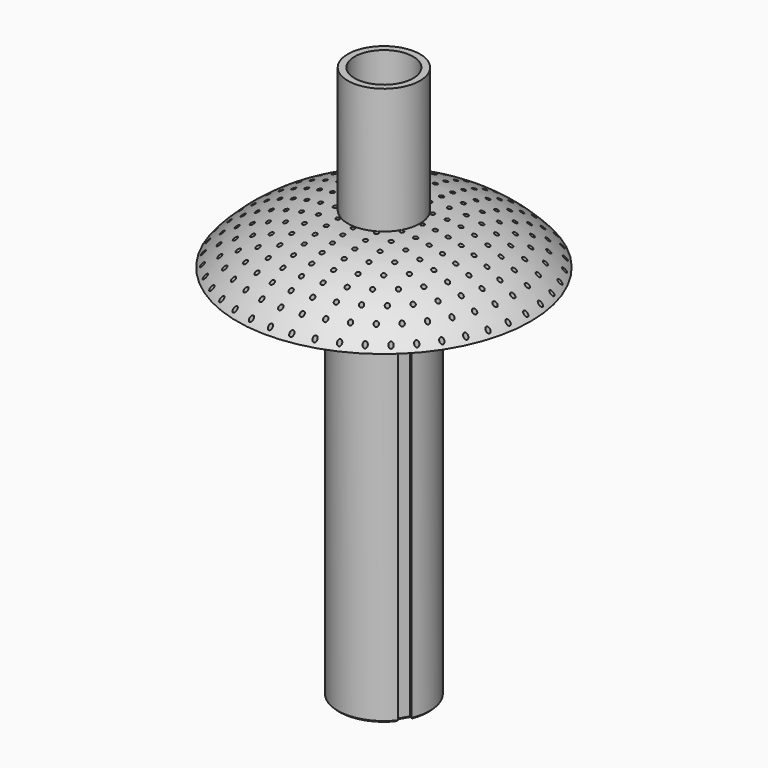
from build123d import *

# Parameters (mm, degrees)
F0_R      = 5.5
F1_DEPTH  = 45
F2_W      = 1.3165529235
F2_H      = 2.0980495028
F3_DEPTH  = 50
F4_R      = 17.5
F5_DEPTH  = 6
F7_R      = 3.5
F8_DEPTH  = 45
F9_SIZE   = 0.2
F11_R     = 0.25
F12_DEPTH = 20.5
F16_DEPTH = 15


# Not quite as in the source:
# - a fillet or chamfer that OpenCascade refuses, or shapes differently, is made with other operations: its cross-section is extruded or revolved along the edge and cut away or added


with BuildPart() as f1:
    # F0 (on Top) → F1 (new body)
    with BuildSketch(Plane.XY):
        Circle(F0_R)
    extrude(amount=F1_DEPTH)

    # F2 (on face) → F3 (cut)
    with BuildSketch(Plane.XY.offset(45)):
        with Locations((0.0565157097, 6.1680867802)):
            Rectangle(F2_W, F2_H)
        Polygon((-4.7906338463, -1.9405028355), (-6.6075980141, -2.9895275869), (-5.9493215523, -4.1296958641), (-4.1323573845, -3.0806711127), align=None)
        Polygon((4.0758416748, -3.1785591934), (5.8928058426, -4.2275839448), (6.5510823044, -3.0874156676), (4.7341181365, -2.0383909162), align=None)
    extrude(amount=-F3_DEPTH, mode=Mode.SUBTRACT)

    # F4 (on face) → F5 (join)
    with BuildSketch(Plane.XY.offset(45)):
        Circle(F4_R)
    extrude(amount=F5_DEPTH)

    # F6: fillet of radius 17.5 on 1 edges, made by hand

    # F6_s1 → F6_t2 (revolve, cut)
    with BuildSketch(Plane.XZ):
        with BuildLine():
            ThreePointArc((17.5, 45), (11.5547824148, 49.4295323221), (4.3090940417, 51))
            Line((4.3090940417, 51), (17.5, 51))
            Line((17.5, 51), (17.5, 45))
        make_face()
    revolve(axis=Axis((0, 0, 51), (0, 0, 1)), mode=Mode.SUBTRACT)

    # F7 (on face) → F8 (cut)
    with BuildSketch(Plane.XY.offset(51)):
        Circle(F7_R)
    extrude(amount=-F8_DEPTH, mode=Mode.SUBTRACT)

    # F9
    f9_edges = [f1.edges().sort_by_distance(p)[0] for p in [
        (4.40498, -2.608475, 0),
        (4.791347, 2.700554, 0),
        (0.714792, 5.286208, 0),
        (0.056516, 5.119062, 0),
        (-0.601761, 5.293022, 0),
        (-4.734422, 2.799151, 0),
        (-4.935387, -2.024076, 0),
        (-4.461496, -2.510587, 0),
        (-4.283011, -3.167651, 0),
        (-0.056925, -5.499705, 0),
        (4.220594, -3.262132, 0),
        (4.884772, -2.125371, 0),
    ]]
    chamfer(f9_edges, length=F9_SIZE)

    # F11 (on offset) → F12 (cut)
    with BuildSketch(Plane.XY.offset(40)):
        with BuildLine():
            ThreePointArc((0, 4.35), (0.1767766953, 4.4232233047), (0.25, 4.6))
            ThreePointArc((0.25, 4.6), (0.1767766953, 4.7767766953), (0, 4.85))
            Line((0, 4.85), (0, 4.35))
        make_face()
        with BuildLine():
            ThreePointArc((0, 6.39), (-0.25, 6.14), (0, 5.89))
            Line((0, 5.89), (0, 6.39))
        make_face()
        with BuildLine():
            Line((0, 6.39), (0, 5.89))
            ThreePointArc((0, 5.89), (0.1767766953, 5.9632233047), (0.25, 6.14))
            ThreePointArc((0.25, 6.14), (0.1767766953, 6.3167766953), (0, 6.39))
        make_face()
        with BuildLine():
            Line((0, 4.35), (0, 4.85))
            ThreePointArc((0, 4.85), (-0.25, 4.6), (0, 4.35))
        make_face()
        with Locations((0, 7.68)):
            Circle(F11_R)
        with Locations((0, 9.22)):
            Circle(F11_R)
        with Locations((0, 10.76)):
            Circle(F11_R)
        with Locations((0, 12.3)):
            Circle(F11_R)
        with Locations((-2.3, 3.9837168574)):
            Circle(F11_R)
        with Locations((-3.9837168574, 2.3)):
            Circle(F11_R)
        with Locations((-4.6, 0)):
            Circle(F11_R)
        with Locations((-3.9837168574, -2.3)):
            Circle(F11_R)
        with Locations((-2.3, -3.9837168574)):
            Circle(F11_R)
        with Locations((0, -4.6)):
            Circle(F11_R)
        with Locations((2.3, -3.9837168574)):
            Circle(F11_R)
        with Locations((3.9837168574, -2.3)):
            Circle(F11_R)
        with Locations((4.6, 0)):
            Circle(F11_R)
        with Locations((3.9837168574, 2.3)):
            Circle(F11_R)
        with Locations((2.3, 3.9837168574)):
            Circle(F11_R)
        with Locations((-2.3496762747, 5.6726203296)):
            Circle(F11_R)
        with Locations((-4.3416356365, 4.3416356365)):
            Circle(F11_R)
        with Locations((-5.6726203296, 2.3496762747)):
            Circle(F11_R)
        with Locations((-6.14, 0)):
            Circle(F11_R)
        with Locations((-5.6726203296, -2.3496762747)):
            Circle(F11_R)
        with Locations((-4.3416356365, -4.3416356365)):
            Circle(F11_R)
        with Locations((-2.3496762747, -5.6726203296)):
            Circle(F11_R)
        with Locations((0, -6.14)):
            Circle(F11_R)
        with Locations((2.3496762747, -5.6726203296)):
            Circle(F11_R)
        with Locations((4.3416356365, -4.3416356365)):
            Circle(F11_R)
        with Locations((5.6726203296, -2.3496762747)):
            Circle(F11_R)
        with Locations((6.14, 0)):
            Circle(F11_R)
        with Locations((5.6726203296, 2.3496762747)):
            Circle(F11_R)
        with Locations((4.3416356365, 4.3416356365)):
            Circle(F11_R)
        with Locations((2.3496762747, 5.6726203296)):
            Circle(F11_R)
        with Locations((-2.3732505168, 7.3041140451)):
            Circle(F11_R)
        with Locations((-4.5141907376, 6.2132505168)):
            Circle(F11_R)
        with Locations((-6.2132505168, 4.5141907376)):
            Circle(F11_R)
        with Locations((-7.3041140451, 2.3732505168)):
            Circle(F11_R)
        with Locations((-7.68, 0)):
            Circle(F11_R)
        with Locations((-7.3041140451, -2.3732505168)):
            Circle(F11_R)
        with Locations((-6.2132505168, -4.5141907376)):
            Circle(F11_R)
        with Locations((-4.5141907376, -6.2132505168)):
            Circle(F11_R)
        with Locations((-2.3732505168, -7.3041140451)):
            Circle(F11_R)
        with Locations((0, -7.68)):
            Circle(F11_R)
        with Locations((2.3732505168, -7.3041140451)):
            Circle(F11_R)
        with Locations((4.5141907376, -6.2132505168)):
            Circle(F11_R)
        with Locations((6.2132505168, -4.5141907376)):
            Circle(F11_R)
        with Locations((7.3041140451, -2.3732505168)):
            Circle(F11_R)
        with Locations((7.68, 0)):
            Circle(F11_R)
        with Locations((7.3041140451, 2.3732505168)):
            Circle(F11_R)
        with Locations((6.2132505168, 4.5141907376)):
            Circle(F11_R)
        with Locations((4.5141907376, 6.2132505168)):
            Circle(F11_R)
        with Locations((2.3732505168, 7.3041140451)):
            Circle(F11_R)
        with Locations((-2.3863115958, 8.9058361184)):
            Circle(F11_R)
        with Locations((-4.61, 7.9847542229)):
            Circle(F11_R)
        with Locations((-6.5195245225, 6.5195245225)):
            Circle(F11_R)
        with Locations((-7.9847542229, 4.61)):
            Circle(F11_R)
        with Locations((-8.9058361184, 2.3863115958)):
            Circle(F11_R)
        with Locations((-9.22, 0)):
            Circle(F11_R)
        with Locations((-8.9058361184, -2.3863115958)):
            Circle(F11_R)
        with Locations((-7.9847542229, -4.61)):
            Circle(F11_R)
        with Locations((-6.5195245225, -6.5195245225)):
            Circle(F11_R)
        with Locations((-4.61, -7.9847542229)):
            Circle(F11_R)
        with Locations((-2.3863115958, -8.9058361184)):
            Circle(F11_R)
        with Locations((0, -9.22)):
            Circle(F11_R)
        with Locations((2.3863115958, -8.9058361184)):
            Circle(F11_R)
        with Locations((4.61, -7.9847542229)):
            Circle(F11_R)
        with Locations((6.5195245225, -6.5195245225)):
            Circle(F11_R)
        with Locations((7.9847542229, -4.61)):
            Circle(F11_R)
        with Locations((8.9058361184, -2.3863115958)):
            Circle(F11_R)
        with Locations((9.22, 0)):
            Circle(F11_R)
        with Locations((8.9058361184, 2.3863115958)):
            Circle(F11_R)
        with Locations((7.9847542229, 4.61)):
            Circle(F11_R)
        with Locations((6.5195245225, 6.5195245225)):
            Circle(F11_R)
        with Locations((4.61, 7.9847542229)):
            Circle(F11_R)
        with Locations((2.3863115958, 8.9058361184)):
            Circle(F11_R)
        with Locations((-2.3943252494, 10.4902243351)):
            Circle(F11_R)
        with Locations((-4.6685890329, 9.6944250186)):
            Circle(F11_R)
        with Locations((-6.708750268, 8.4125067514)):
            Circle(F11_R)
        with Locations((-8.4125067514, 6.708750268)):
            Circle(F11_R)
        with Locations((-9.6944250186, 4.6685890329)):
            Circle(F11_R)
        with Locations((-10.4902243351, 2.3943252494)):
            Circle(F11_R)
        with Locations((-10.76, 0)):
            Circle(F11_R)
        with Locations((-10.4902243351, -2.3943252494)):
            Circle(F11_R)
        with Locations((-9.6944250186, -4.6685890329)):
            Circle(F11_R)
        with Locations((-8.4125067514, -6.708750268)):
            Circle(F11_R)
        with Locations((-6.708750268, -8.4125067514)):
            Circle(F11_R)
        with Locations((-4.6685890329, -9.6944250186)):
            Circle(F11_R)
        with Locations((-2.3943252494, -10.4902243351)):
            Circle(F11_R)
        with Locations((0, -10.76)):
            Circle(F11_R)
        with Locations((2.3943252494, -10.4902243351)):
            Circle(F11_R)
        with Locations((4.6685890329, -9.6944250186)):
            Circle(F11_R)
        with Locations((6.708750268, -8.4125067514)):
            Circle(F11_R)
        with Locations((8.4125067514, -6.708750268)):
            Circle(F11_R)
        with Locations((9.6944250186, -4.6685890329)):
            Circle(F11_R)
        with Locations((10.4902243351, -2.3943252494)):
            Circle(F11_R)
        with Locations((10.76, 0)):
            Circle(F11_R)
        with Locations((10.4902243351, 2.3943252494)):
            Circle(F11_R)
        with Locations((9.6944250186, 4.6685890329)):
            Circle(F11_R)
        with Locations((8.4125067514, 6.708750268)):
            Circle(F11_R)
        with Locations((6.708750268, 8.4125067514)):
            Circle(F11_R)
        with Locations((4.6685890329, 9.6944250186)):
            Circle(F11_R)
        with Locations((2.3943252494, 10.4902243351)):
            Circle(F11_R)
        with Locations((-2.3996109608, 12.063658949)):
            Circle(F11_R)
        with Locations((-4.7070062181, 11.3637182499)):
            Circle(F11_R)
        with Locations((-6.8335138661, 10.2270762313)):
            Circle(F11_R)
        with Locations((-8.6974134086, 8.6974134086)):
            Circle(F11_R)
        with Locations((-10.2270762313, 6.8335138661)):
            Circle(F11_R)
        with Locations((-11.3637182499, 4.7070062181)):
            Circle(F11_R)
        with Locations((-12.063658949, 2.3996109608)):
            Circle(F11_R)
        with Locations((-12.3, 0)):
            Circle(F11_R)
        with Locations((-12.063658949, -2.3996109608)):
            Circle(F11_R)
        with Locations((-11.3637182499, -4.7070062181)):
            Circle(F11_R)
        with Locations((-10.2270762313, -6.8335138661)):
            Circle(F11_R)
        with Locations((-8.6974134086, -8.6974134086)):
            Circle(F11_R)
        with Locations((-6.8335138661, -10.2270762313)):
            Circle(F11_R)
        with Locations((-4.7070062181, -11.3637182499)):
            Circle(F11_R)
        with Locations((-2.3996109608, -12.063658949)):
            Circle(F11_R)
        with Locations((0, -12.3)):
            Circle(F11_R)
        with Locations((2.3996109608, -12.063658949)):
            Circle(F11_R)
        with Locations((4.7070062181, -11.3637182499)):
            Circle(F11_R)
        with Locations((6.8335138661, -10.2270762313)):
            Circle(F11_R)
        with Locations((8.6974134086, -8.6974134086)):
            Circle(F11_R)
        with Locations((10.2270762313, -6.8335138661)):
            Circle(F11_R)
        with Locations((11.3637182499, -4.7070062181)):
            Circle(F11_R)
        with Locations((12.063658949, -2.3996109608)):
            Circle(F11_R)
        with Locations((12.3, 0)):
            Circle(F11_R)
        with Locations((12.063658949, 2.3996109608)):
            Circle(F11_R)
        with Locations((11.3637182499, 4.7070062181)):
            Circle(F11_R)
        with Locations((10.2270762313, 6.8335138661)):
            Circle(F11_R)
        with Locations((8.6974134086, 8.6974134086)):
            Circle(F11_R)
        with Locations((6.8335138661, 10.2270762313)):
            Circle(F11_R)
        with Locations((4.7070062181, 11.3637182499)):
            Circle(F11_R)
        with Locations((2.3996109608, 12.063658949)):
            Circle(F11_R)
        with Locations((0, 13.84)):
            Circle(F11_R)
        with Locations((0, 15.38)):
            Circle(F11_R)
        with Locations((0, 16.92)):
            Circle(F11_R)
        with Locations((-2.4032907789, 13.6297393017)):
            Circle(F11_R)
        with Locations((-4.7335587836, 13.0053458717)):
            Circle(F11_R)
        with Locations((-6.92, 11.9857915884)):
            Circle(F11_R)
        with Locations((-8.8961805181, 10.6020550928)):
            Circle(F11_R)
        with Locations((-10.6020550928, 8.8961805181)):
            Circle(F11_R)
        with Locations((-11.9857915884, 6.92)):
            Circle(F11_R)
        with Locations((-13.0053458717, 4.7335587836)):
            Circle(F11_R)
        with Locations((-13.6297393017, 2.4032907789)):
            Circle(F11_R)
        with Locations((-13.84, 0)):
            Circle(F11_R)
        with Locations((-13.6297393017, -2.4032907789)):
            Circle(F11_R)
        with Locations((-13.0053458717, -4.7335587836)):
            Circle(F11_R)
        with Locations((-11.9857915884, -6.92)):
            Circle(F11_R)
        with Locations((-10.6020550928, -8.8961805181)):
            Circle(F11_R)
        with Locations((-8.8961805181, -10.6020550928)):
            Circle(F11_R)
        with Locations((-6.92, -11.9857915884)):
            Circle(F11_R)
        with Locations((-4.7335587836, -13.0053458717)):
            Circle(F11_R)
        with Locations((-2.4032907789, -13.6297393017)):
            Circle(F11_R)
        with Locations((0, -13.84)):
            Circle(F11_R)
        with Locations((2.4032907789, -13.6297393017)):
            Circle(F11_R)
        with Locations((4.7335587836, -13.0053458717)):
            Circle(F11_R)
        with Locations((6.92, -11.9857915884)):
            Circle(F11_R)
        with Locations((8.8961805181, -10.6020550928)):
            Circle(F11_R)
        with Locations((10.6020550928, -8.8961805181)):
            Circle(F11_R)
        with Locations((11.9857915884, -6.92)):
            Circle(F11_R)
        with Locations((13.0053458717, -4.7335587836)):
            Circle(F11_R)
        with Locations((13.6297393017, -2.4032907789)):
            Circle(F11_R)
        with Locations((13.84, 0)):
            Circle(F11_R)
        with Locations((13.6297393017, 2.4032907789)):
            Circle(F11_R)
        with Locations((13.0053458717, 4.7335587836)):
            Circle(F11_R)
        with Locations((11.9857915884, 6.92)):
            Circle(F11_R)
        with Locations((10.6020550928, 8.8961805181)):
            Circle(F11_R)
        with Locations((8.8961805181, 10.6020550928)):
            Circle(F11_R)
        with Locations((6.92, 11.9857915884)):
            Circle(F11_R)
        with Locations((4.7335587836, 13.0053458717)):
            Circle(F11_R)
        with Locations((2.4032907789, 13.6297393017)):
            Circle(F11_R)
        with Locations((-2.4059620723, 15.1906466784)):
            Circle(F11_R)
        with Locations((-4.7526813735, 14.6272492206)):
            Circle(F11_R)
        with Locations((-6.982373886, 13.703680342)):
            Circle(F11_R)
        with Locations((-9.0401371803, 12.4426813735)):
            Circle(F11_R)
        with Locations((-10.8753022946, 10.8753022946)):
            Circle(F11_R)
        with Locations((-12.4426813735, 9.0401371803)):
            Circle(F11_R)
        with Locations((-13.703680342, 6.982373886)):
            Circle(F11_R)
        with Locations((-14.6272492206, 4.7526813735)):
            Circle(F11_R)
        with Locations((-15.1906466784, 2.4059620723)):
            Circle(F11_R)
        with Locations((-15.38, 0)):
            Circle(F11_R)
        with Locations((-15.1906466784, -2.4059620723)):
            Circle(F11_R)
        with Locations((-14.6272492206, -4.7526813735)):
            Circle(F11_R)
        with Locations((-13.703680342, -6.982373886)):
            Circle(F11_R)
        with Locations((-12.4426813735, -9.0401371803)):
            Circle(F11_R)
        with Locations((-10.8753022946, -10.8753022946)):
            Circle(F11_R)
        with Locations((-9.0401371803, -12.4426813735)):
            Circle(F11_R)
        with Locations((-6.982373886, -13.703680342)):
            Circle(F11_R)
        with Locations((-4.7526813735, -14.6272492206)):
            Circle(F11_R)
        with Locations((-2.4059620723, -15.1906466784)):
            Circle(F11_R)
        with Locations((0, -15.38)):
            Circle(F11_R)
        with Locations((2.4059620723, -15.1906466784)):
            Circle(F11_R)
        with Locations((4.7526813735, -14.6272492206)):
            Circle(F11_R)
        with Locations((6.982373886, -13.703680342)):
            Circle(F11_R)
        with Locations((9.0401371803, -12.4426813735)):
            Circle(F11_R)
        with Locations((10.8753022946, -10.8753022946)):
            Circle(F11_R)
        with Locations((12.4426813735, -9.0401371803)):
            Circle(F11_R)
        with Locations((13.703680342, -6.982373886)):
            Circle(F11_R)
        with Locations((14.6272492206, -4.7526813735)):
            Circle(F11_R)
        with Locations((15.1906466784, -2.4059620723)):
            Circle(F11_R)
        with Locations((15.38, 0)):
            Circle(F11_R)
        with Locations((15.1906466784, 2.4059620723)):
            Circle(F11_R)
        with Locations((14.6272492206, 4.7526813735)):
            Circle(F11_R)
        with Locations((13.703680342, 6.982373886)):
            Circle(F11_R)
        with Locations((12.4426813735, 9.0401371803)):
            Circle(F11_R)
        with Locations((10.8753022946, 10.8753022946)):
            Circle(F11_R)
        with Locations((9.0401371803, 12.4426813735)):
            Circle(F11_R)
        with Locations((6.982373886, 13.703680342)):
            Circle(F11_R)
        with Locations((4.7526813735, 14.6272492206)):
            Circle(F11_R)
        with Locations((2.4059620723, 15.1906466784)):
            Circle(F11_R)
        with Locations((-2.4079670636, 16.7477787966)):
            Circle(F11_R)
        with Locations((-4.7669148618, 16.2346211136)):
            Circle(F11_R)
        with Locations((-7.02882202, 15.3909733614)):
            Circle(F11_R)
        with Locations((-9.1476426313, 14.2340097755)):
            Circle(F11_R)
        with Locations((-11.0802436184, 12.7872827981)):
            Circle(F11_R)
        with Locations((-12.7872827981, 11.0802436184)):
            Circle(F11_R)
        with Locations((-14.2340097755, 9.1476426313)):
            Circle(F11_R)
        with Locations((-15.3909733614, 7.02882202)):
            Circle(F11_R)
        with Locations((-16.2346211136, 4.7669148618)):
            Circle(F11_R)
        with Locations((-16.7477787966, 2.4079670636)):
            Circle(F11_R)
        with Locations((-16.92, 0)):
            Circle(F11_R)
        with Locations((-16.7477787966, -2.4079670636)):
            Circle(F11_R)
        with Locations((-16.2346211136, -4.7669148618)):
            Circle(F11_R)
        with Locations((-15.3909733614, -7.02882202)):
            Circle(F11_R)
        with Locations((-14.2340097755, -9.1476426313)):
            Circle(F11_R)
        with Locations((-12.7872827981, -11.0802436184)):
            Circle(F11_R)
        with Locations((-11.0802436184, -12.7872827981)):
            Circle(F11_R)
        with Locations((-9.1476426313, -14.2340097755)):
            Circle(F11_R)
        with Locations((-7.02882202, -15.3909733614)):
            Circle(F11_R)
        with Locations((-4.7669148618, -16.2346211136)):
            Circle(F11_R)
        with Locations((-2.4079670636, -16.7477787966)):
            Circle(F11_R)
        with Locations((0, -16.92)):
            Circle(F11_R)
        with Locations((2.4079670636, -16.7477787966)):
            Circle(F11_R)
        with Locations((4.7669148618, -16.2346211136)):
            Circle(F11_R)
        with Locations((7.02882202, -15.3909733614)):
            Circle(F11_R)
        with Locations((9.1476426313, -14.2340097755)):
            Circle(F11_R)
        with Locations((11.0802436184, -12.7872827981)):
            Circle(F11_R)
        with Locations((12.7872827981, -11.0802436184)):
            Circle(F11_R)
        with Locations((14.2340097755, -9.1476426313)):
            Circle(F11_R)
        with Locations((15.3909733614, -7.02882202)):
            Circle(F11_R)
        with Locations((16.2346211136, -4.7669148618)):
            Circle(F11_R)
        with Locations((16.7477787966, -2.4079670636)):
            Circle(F11_R)
        with Locations((16.92, 0)):
            Circle(F11_R)
        with Locations((16.7477787966, 2.4079670636)):
            Circle(F11_R)
        with Locations((16.2346211136, 4.7669148618)):
            Circle(F11_R)
        with Locations((15.3909733614, 7.02882202)):
            Circle(F11_R)
        with Locations((14.2340097755, 9.1476426313)):
            Circle(F11_R)
        with Locations((12.7872827981, 11.0802436184)):
            Circle(F11_R)
        with Locations((11.0802436184, 12.7872827981)):
            Circle(F11_R)
        with Locations((9.1476426313, 14.2340097755)):
            Circle(F11_R)
        with Locations((7.02882202, 15.3909733614)):
            Circle(F11_R)
        with Locations((4.7669148618, 16.2346211136)):
            Circle(F11_R)
        with Locations((2.4079670636, 16.7477787966)):
            Circle(F11_R)
    extrude(amount=F12_DEPTH, mode=Mode.SUBTRACT)

    # F13 (on Right) → F15 (revolve, cut)
    with BuildSketch(Plane.YZ):
        with BuildLine():
            Line((5.5, 49), (5.5, 45))
            Line((5.5, 45), (15, 45))
            ThreePointArc((15, 45), (10.5739891785, 47.7694742989), (5.5, 49))
        make_face()
    revolve(axis=Axis((0, 0, 17.0523002744), (0, 0, 1)), mode=Mode.SUBTRACT)

    # F16 (add): a face of the model
    f16_faces = [f1.faces().sort_by_distance(p)[0] for p in [
        (-4.187214457, 0, 51),
    ]]
    extrude(f16_faces, amount=F16_DEPTH)


solid = f1.part
